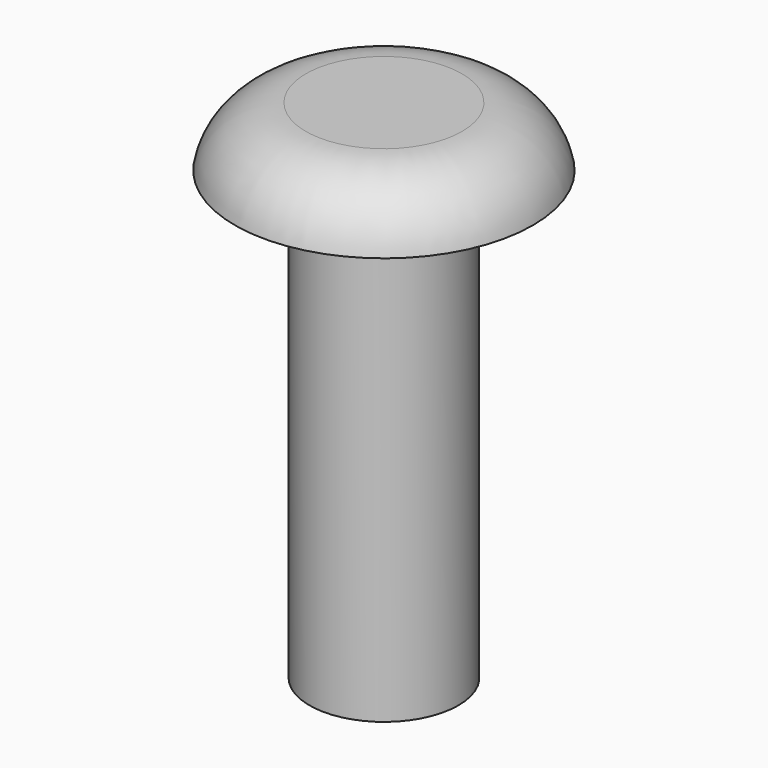
from build123d import *

# Parameters (mm, degrees)
F0_R     = 6.35
F1_DEPTH = 2.54
F3_R     = 3.175
F4_DEPTH = 19.05


# Not quite as in the source:
# - a fillet or chamfer that OpenCascade refuses, or shapes differently, is made with other operations: its cross-section is extruded or revolved along the edge and cut away or added


with BuildPart() as f1:
    # F0 (on Top) → F1 (new body)
    with BuildSketch(Plane.XY):
        Circle(F0_R)
    extrude(amount=F1_DEPTH)

    # F2: fillet of radius 3.0660512242 on 1 edges, made by hand

    # F2_s1 → F2_t2 (revolve, cut)
    with BuildSketch(Plane.XZ):
        with BuildLine():
            ThreePointArc((6.35, 0), (5.3027068749, 1.8206027884), (3.3294139279, 2.54))
            Line((3.3294139279, 2.54), (6.35, 2.54))
            Line((6.35, 2.54), (6.35, 0))
        make_face()
    revolve(axis=Axis((0, 0, 2.54), (0, 0, 1)), mode=Mode.SUBTRACT)

    # F3 (on face) → F4 (join)
    with BuildSketch(Plane(origin=(0, 0, 0), x_dir=(1, 0, 0), z_dir=(0, 0, -1))):
        Circle(F3_R)
    extrude(amount=F4_DEPTH)


solid = f1.part
